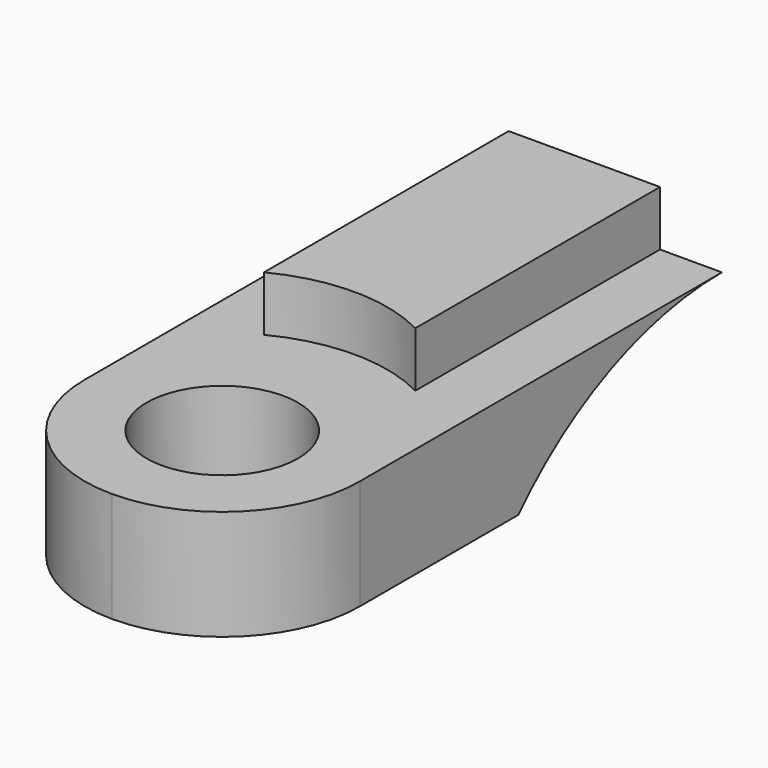
from build123d import *

# Parameters (mm, degrees)
F1_DEPTH = 5
F2_R     = 2.75
F3_DEPTH = 4.001
F4_R     = 4.99999
F6_DEPTH = 2


# Not quite as in the source:
# - a fillet or chamfer is up to 0.001 mm smaller than in the source, because OpenCascade refuses the exact size


with BuildPart() as f1:
    # F0 (on Right) → F1 (new body, symmetric)
    with BuildSketch(Plane.YZ):
        with BuildLine():
            Line((16.45, 0), (0, 0))
            Line((0, 0), (-5, 0))
            Line((-5, 0), (-5, -4))
            Line((-5, -4), (7.197973195, -4))
            ThreePointArc((7.197973195, -4), (11.4101587327, -1.0428133754), (16.45, 0))
        make_face()
    extrude(amount=F1_DEPTH, both=True)

    # F2 (on face) → F3 (cut, through all)
    with BuildSketch(Plane.XY):
        Circle(F2_R)
    extrude(amount=-F3_DEPTH, mode=Mode.SUBTRACT)

    # F4 (radius 5 in the source; OpenCascade refuses exactly that, so slightly less here)
    f4_edges = [f1.edges().sort_by_distance(p)[0] for p in [
        (5, -5, -2),
        (-5, -5, -2),
    ]]
    fillet(f4_edges, radius=F4_R)

    # F5 (on face) → F6 (join)
    with BuildSketch(Plane.XY):
        with BuildLine():
            Line((-2.75, 16.45), (-2.75, 5.3326822519))
            ThreePointArc((-2.75, 5.3326822519), (0, 6), (2.75, 5.3326822519))
            Line((2.75, 5.3326822519), (2.75, 16.45))
            Line((2.75, 16.45), (-2.75, 16.45))
        make_face()
    extrude(amount=F6_DEPTH)


solid = f1.part
